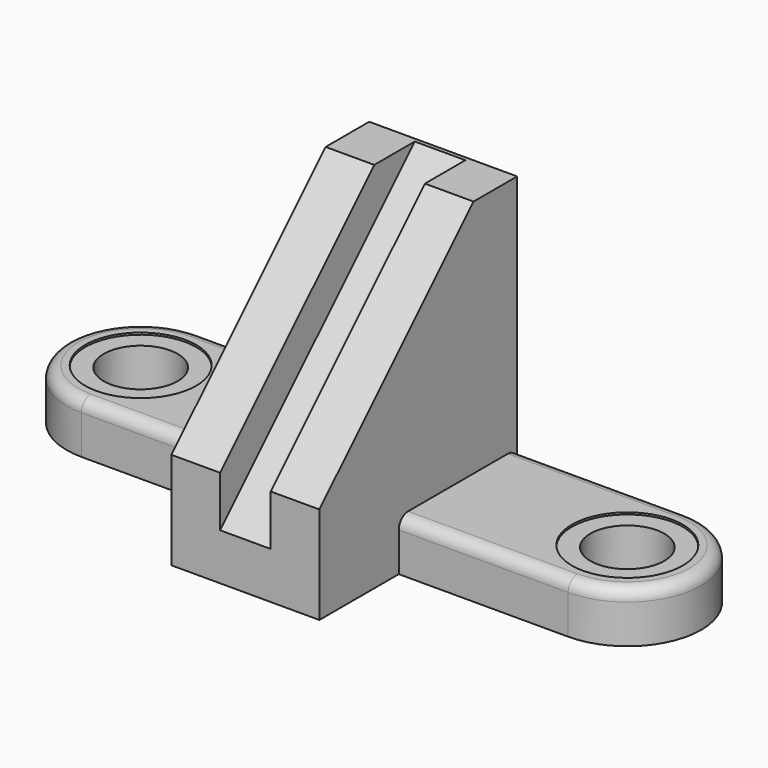
from build123d import *

# Parameters (mm, degrees)
F1_DEPTH = 38
F3_DEPTH = 13
F5_DEPTH = 26
F6_R     = 28.5
F7_DEPTH = 1
F8_R     = 19
F9_DEPTH = 25
F10_R    = 6


# Not quite as in the source:
# - a pattern or mirror of a feature is missing from the dataset's text; its kind, count and spacing are read off the source's solid


with BuildPart() as f1:
    # F0 (on Right) → F1 (new body, symmetric)
    with BuildSketch(Plane.YZ):
        Polygon((-127, 0), (0, 0), (0, 149), (-28, 149), (-127, 50), align=None)
    extrude(amount=F1_DEPTH, both=True)

    # F2 (on Right) → F3 (cut, symmetric)
    with BuildSketch(Plane.YZ):
        Polygon((-127, 24), (-2, 149), (-28, 149), (-127, 50), align=None)
    extrude(amount=F3_DEPTH, both=True, mode=Mode.SUBTRACT)

    # F4 (on Top) → F5 (join)
    with BuildSketch(Plane.XY):
        with BuildLine():
            ThreePointArc((-125, 0), (-163, -38), (-125, -76))
            Line((-125, -76), (125, -76))
            ThreePointArc((125, -76), (163, -38), (125, 0))
            Line((125, 0), (-125, 0))
        make_face()
    extrude(amount=F5_DEPTH)

    # F6 (on face) → F7 (cut)
    with BuildSketch(Plane.XY.offset(26)):
        with Locations((-125, -38)):
            Circle(F6_R)
    f7 = extrude(amount=-F7_DEPTH, mode=Mode.SUBTRACT)

    # F7_copies: F7 across plane
    add(f7.mirror(Plane(origin=(0, 0, 0), x_dir=(0, 0, 1), z_dir=(1, 0, 0))), mode=Mode.SUBTRACT)

    # F8 (on face) → F9 (cut, through all)
    with BuildSketch(Plane.XY.offset(25)):
        with Locations((-125, -38)):
            Circle(F8_R)
    f9 = extrude(amount=-F9_DEPTH, mode=Mode.SUBTRACT)

    # F9_copies: F9 across plane
    add(f9.mirror(Plane(origin=(0, 0, 0), x_dir=(0, 0, 1), z_dir=(1, 0, 0))), mode=Mode.SUBTRACT)

    # F10
    f10_edges = [f1.edges().sort_by_distance(p)[0] for p in [
        (-81.5, -76, 26),
        (81.5, 0, 26),
        (81.5, -76, 26),
        (163, -38, 26),
        (-163, -38, 26),
        (-81.5, 0, 26),
    ]]
    fillet(f10_edges, radius=F10_R)


solid = f1.part
